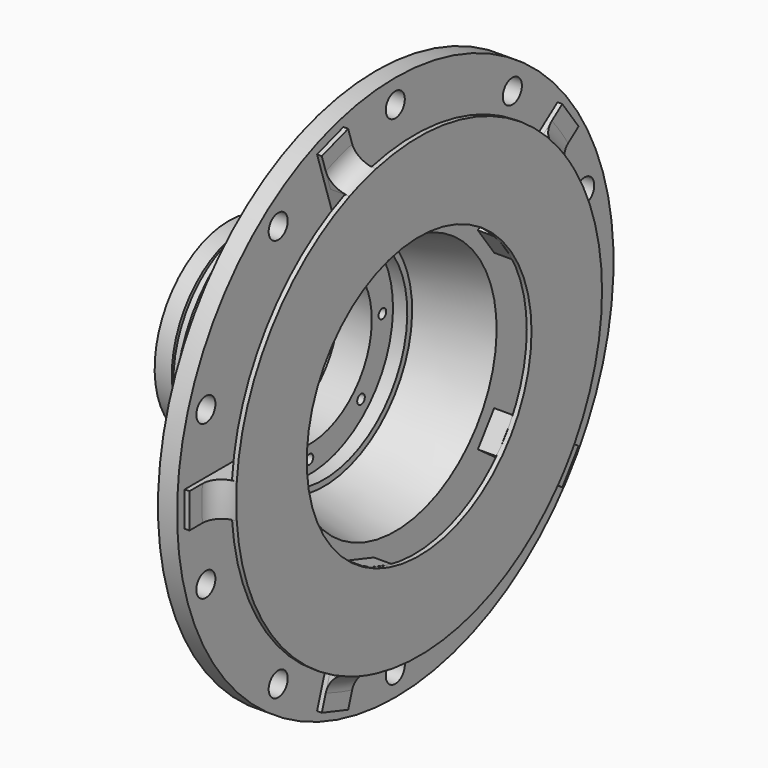
from build123d import *

# Parameters (mm, degrees)
F2_R          = 12.5
F3_DEPTH      = 20
F4_R          = 5
F5_DEPTH      = 20
F6_W          = 129.0251463652
F6_H          = 36.3384204739
F7_DEPTH      = 20
F9_DEPTH      = 5
F10_DEPTH     = 15
F11_T4_ANGLE  = 32.5973484346
F11_T10_ANGLE = 32.5973484346
F11_T16_ANGLE = 32.5973484346
F11_T22_ANGLE = 32.5973484346
F11_T28_ANGLE = 32.5973484346


# Not quite as in the source:
# - a fillet or chamfer that OpenCascade refuses, or shapes differently, is made with other operations: its cross-section is extruded or revolved along the edge and cut away or added


with BuildPart() as f1:
    # F0 (on Front) → F1 (revolve)
    with BuildSketch(Plane.XZ):
        with BuildLine():
            Line((-16.3140908403, 189.203946461), (-16.3140908403, 151.1775321185))
            Line((-16.3140908403, 151.1775321185), (-41.3140908403, 136.1826956272))
            Line((-41.3140908403, 136.1826956272), (-41.3140908403, 124.7942986206))
            Line((-41.3140908403, 124.7942986206), (-111.3140908403, 106.3929200172))
            Line((-111.3140908403, 106.3929200172), (-110.7086323423, 106.3929200172))
            Line((-110.7086323423, 106.3929200172), (-110.7086323423, 103.5716161132))
            Line((-110.7086323423, 103.5716161132), (-117.2448031826, 103.5716161132))
            Line((-117.2448031826, 103.5716161132), (-117.2448031826, 100.1479104161))
            Line((-117.2448031826, 100.1479104161), (-110.7086323423, 100.1479104161))
            Line((-110.7086323423, 100.1479104161), (-110.7086323423, 94.2342355847))
            Line((-110.7086323423, 94.2342355847), (-117.2448031826, 94.2342355847))
            Line((-117.2448031826, 94.2342355847), (-117.2448031826, 82.7181264758))
            Line((-117.2448031826, 82.7181264758), (-123.3140908403, 76.9600793719))
            Line((-123.3140908403, 76.9600793719), (-141.3140908403, 76.9600793719))
            Line((-141.3140908403, 76.9600793719), (-148.0058894081, 70.7351565361))
            Line((-148.0058894081, 70.7351565361), (-165.9934520721, 70.7351565361))
            Line((-165.9934520721, 70.7351565361), (-165.9934520721, 41.6837670207))
            Line((-165.9934520721, 41.6837670207), (-147.6857364697, 41.6837670207))
            Line((-147.6857364697, 41.6837670207), (-138.2742375655, 47.9580983818))
            Line((-138.2742375655, 47.9580983818), (-124.5491505189, 47.9580983818))
            Line((-124.5491505189, 47.9580983818), (-116.3140908403, 55.3639903963))
            Line((-116.3140908403, 55.3639903963), (-81.3140908403, 55.3639903963))
            Line((-81.3140908403, 55.3639903963), (-81.3140908403, 83.1748159732))
            Line((-81.3140908403, 83.1748159732), (-66.3140908403, 83.1748159732))
            Line((-66.3140908403, 83.1748159732), (-66.3140908403, 89.5191647847))
            Line((-66.3140908403, 89.5191647847), (8.6859091597, 106.4794477311))
            Line((8.6859091597, 106.4794477311), (8.6859091597, 259.7348150386))
            Line((8.6859091597, 259.7348150386), (-11.3140908403, 259.7348150386))
            Line((-11.3140908403, 259.7348150386), (-11.3140908403, 209.7348150386))
            Line((-11.3140908403, 209.7348150386), (-41.3140908403, 209.7348150386))
            Line((-41.3140908403, 209.7348150386), (-41.3140908403, 203.7348150386))
            Line((-41.3140908403, 203.7348150386), (-23.6449593669, 198.8411523412))
            ThreePointArc((-23.6449593669, 198.8411523412), (-18.355092325, 195.25822946), (-16.3140908403, 189.203946461))
        make_face()
    revolve(axis=Axis((-78.6537714562, 0, -26.3162329793), (-1, 0, 0)))

    # F2 (on face) → F3 (cut)
    with BuildSketch(Plane(origin=(-11.3140908403, 0, 0), x_dir=(0, -1, 0), z_dir=(-1, 0, 0))):
        with Locations((0, 234.7348150386)):
            Circle(F2_R)
        with Locations((-153.4419561204, 184.8785012666)):
            Circle(F2_R)
        with Locations((-248.2743003031, 54.3529772576)):
            Circle(F2_R)
        with Locations((-248.2743003031, -106.9854432162)):
            Circle(F2_R)
        with Locations((-153.4419561204, -237.5109672252)):
            Circle(F2_R)
        with Locations((0, -287.3672809972)):
            Circle(F2_R)
        with Locations((153.4419561204, -237.5109672252)):
            Circle(F2_R)
        with Locations((248.2743003031, -106.9854432162)):
            Circle(F2_R)
        with Locations((248.2743003031, 54.3529772576)):
            Circle(F2_R)
        with Locations((153.4419561204, 184.8785012666)):
            Circle(F2_R)
    extrude(amount=-F3_DEPTH, mode=Mode.SUBTRACT)

    # F4 (on face) → F5 (cut)
    with BuildSketch(Plane.YZ.offset(-81.3140908403)):
        with Locations((0, 69.2694031847)):
            Circle(F4_R)
        with Locations((-67.5892515156, 41.2730185363)):
            Circle(F4_R)
        with Locations((-95.585636164, -26.3162329793)):
            Circle(F4_R)
        with Locations((-67.5892515156, -93.9054844949)):
            Circle(F4_R)
        with Locations((0, -121.9018691433)):
            Circle(F4_R)
        with Locations((67.5892515156, -93.9054844949)):
            Circle(F4_R)
        with Locations((95.585636164, -26.3162329793)):
            Circle(F4_R)
        with Locations((67.5892515156, 41.2730185363)):
            Circle(F4_R)
    extrude(amount=-F5_DEPTH, mode=Mode.SUBTRACT)

    # F6 (on face) → F7 (join)
    with BuildSketch(Plane.YZ.offset(8.6859091597)):
        with Locations((-211.5166261792, -26.3162329793)):
            Rectangle(F6_W, F6_H)
        Polygon((-102.5776593383, -283.2210069825), (-68.0177677547, -294.4501964577), (-28.1468048262, -171.7399902411), (-62.7066964097, -160.510800766), align=None)
        Polygon((212.6327194043, -203.2613254223), (233.9919070505, -173.8629257102), (129.6083709393, -98.0238475019), (108.2491832932, -127.422247214), align=None)
        Polygon((233.9919070505, 121.2304597516), (212.6327194043, 150.6288594637), (108.2491832932, 74.7897812554), (129.6083709393, 45.3913815433), align=None)
        Polygon((-68.0177677547, 241.8177304991), (-102.5776593383, 230.5885410239), (-62.7066964097, 107.8783348074), (-28.1468048262, 119.1075242825), align=None)
    extrude(amount=F7_DEPTH)

    # F8 (on face) → F9 (join)
    with BuildSketch(Plane.YZ.offset(28.6859091597)):
        with BuildLine():
            Line((-147.0040529966, -8.1470227424), (-239.0119979178, -8.1470227424))
            ThreePointArc((-239.0119979178, -8.1470227424), (-239.701596468, -26.3162329793), (-239.0119979178, -44.4854432162))
            Line((-239.0119979178, -44.4854432162), (-147.0040529966, -44.4854432162))
            Line((-147.0040529966, -44.4854432162), (-147.0040529966, -35.9564862394))
            ThreePointArc((-147.0040529966, -35.9564862394), (-147.3198088526, -26.3162329793), (-147.0040529966, -16.6759797192))
            Line((-147.0040529966, -16.6759797192), (-147.0040529966, -8.1470227424))
        make_face()
        with BuildLine():
            ThreePointArc((-239.0119979178, -44.4854432162), (9.0911460608, -265.8453677679), (239.701596468, -26.3162329793))
            ThreePointArc((239.701596468, -26.3162329793), (9.0911460608, 213.2129018093), (-239.0119979178, -8.1470227424))
            Line((-239.0119979178, -8.1470227424), (-147.0040529966, -8.1470227424))
            Line((-147.0040529966, -8.1470227424), (-147.0040529966, -16.6759797192))
            ThreePointArc((-147.0040529966, -16.6759797192), (4.8227114956, 120.9246157489), (147.3198088526, -26.3162329793))
            ThreePointArc((147.3198088526, -26.3162329793), (4.8227114956, -173.5570817074), (-147.0040529966, -35.9564862394))
            Line((-147.0040529966, -35.9564862394), (-147.0040529966, -44.4854432162))
            Line((-147.0040529966, -44.4854432162), (-239.0119979178, -44.4854432162))
        make_face()
    extrude(amount=F9_DEPTH)

    # F10 (cut): faces of the model
    f10_faces = [f1.faces().sort_by_distance(p)[0] for p in [
        (28.6859091597, -79.6491158165, -271.4510054782),
        (28.6859091597, -257.7499531299, -26.3162329793),
        (28.6859091597, 208.5240923814, -177.8178542081),
        (28.6859091597, -79.6491158165, 218.8185395196),
        (28.6859091597, 208.5240923814, 125.1853882495),
    ]]
    extrude(f10_faces, amount=-F10_DEPTH, mode=Mode.SUBTRACT)

    # F11: fillet of radius 20 on 5 edges, made by hand


with BuildPart() as f11_tool2:
    # F11_s3 → F11_t4 (revolve)
    with BuildSketch(Plane(origin=(0, -7.0886957411, -24.2435313329), x_dir=(1, 0, 0), z_dir=(0, 0.2806444996, 0.9598117861))):
        with BuildLine():
            ThreePointArc((13.6859091597, -252.3160904308), (19.5437735359, -238.1739548071), (33.6859091597, -232.3160904308))
            Line((33.6859091597, -232.3160904308), (33.6859091597, -231.9160904308))
            Line((33.6859091597, -231.9160904308), (13.2859091597, -231.9160904308))
            Line((13.2859091597, -231.9160904308), (13.2859091597, -252.3160904308))
            Line((13.2859091597, -252.3160904308), (13.6859091597, -252.3160904308))
        make_face()
    revolve(axis=Axis((13.6859091597, 0, -26.3162329793), (1, 0, 0)), revolution_arc=F11_T4_ANGLE)

    split(bisect_by=Plane.XY.offset(-44.4854432162), keep=Keep.TOP)

    split(bisect_by=Plane.XY.offset(-8.1470227424), keep=Keep.BOTTOM)


with BuildPart() as f1_1:
    add(f1.part)

    # F11_t1: union F11_tool2
    add(f11_tool2.part)


with BuildPart() as f11_tool8:
    # F11_s9 → F11_t10 (revolve)
    with BuildSketch(Plane(origin=(0, -0.7809680379, -0.0231966772), x_dir=(1, 0, 0), z_dir=(0, 0.9995591734, 0.0296893732))):
        with BuildLine():
            ThreePointArc((13.6859091597, -233.3969643843), (19.5437735359, -219.2548287605), (33.6859091597, -213.3969643843))
            Line((33.6859091597, -213.3969643843), (33.6859091597, -212.9969643843))
            Line((33.6859091597, -212.9969643843), (13.2859091597, -212.9969643843))
            Line((13.2859091597, -212.9969643843), (13.2859091597, -233.3969643843))
            Line((13.2859091597, -233.3969643843), (13.6859091597, -233.3969643843))
        make_face()
    revolve(axis=Axis((13.6859091597, 0, -26.3162329793), (1, 0, 0)), revolution_arc=F11_T10_ANGLE)

    split(bisect_by=Plane(origin=(0, 9.5457989712, 3.101618102), x_dir=(1, 0, 0), z_dir=(0, -0.9510565163, -0.3090169944)), keep=Keep.TOP)

    split(bisect_by=Plane(origin=(0, -25.0140926123, -8.1275713731), x_dir=(1, 0, 0), z_dir=(0, 0.9510565163, 0.3090169944)), keep=Keep.TOP)


with BuildPart() as f1_2:
    add(f1_1.part)

    # F11_t7: union F11_tool8
    add(f11_tool8.part)


with BuildPart() as f11_tool14:
    # F11_s15 → F11_t16 (revolve)
    with BuildSketch(Plane(origin=(0, 12.2507186828, -8.3564583064), x_dir=(1, 0, 0), z_dir=(0, -0.8261113339, 0.5635069335))):
        with BuildLine():
            ThreePointArc((13.6859091597, -281.4417347966), (19.5437735359, -267.2995991729), (33.6859091597, -261.4417347966))
            Line((33.6859091597, -261.4417347966), (33.6859091597, -261.0417347966))
            Line((33.6859091597, -261.0417347966), (13.2859091597, -261.0417347966))
            Line((13.2859091597, -261.0417347966), (13.2859091597, -281.4417347966))
            Line((13.2859091597, -281.4417347966), (13.6859091597, -281.4417347966))
        make_face()
    revolve(axis=Axis((13.6859091597, 0, -26.3162329793), (1, 0, 0)), revolution_arc=F11_T16_ANGLE)

    split(bisect_by=Plane(origin=(0, 25.0140926123, -8.1275713731), x_dir=(1, 0, 0), z_dir=(0, -0.9510565163, 0.3090169944)), keep=Keep.TOP)

    split(bisect_by=Plane(origin=(0, -9.5457989712, 3.101618102), x_dir=(1, 0, 0), z_dir=(0, 0.9510565163, -0.3090169944)), keep=Keep.TOP)


with BuildPart() as f1_3:
    add(f1_2.part)

    # F11_t13: union F11_tool14
    add(f11_tool14.part)


with BuildPart() as f11_tool20:
    # F11_s21 → F11_t22 (revolve)
    with BuildSketch(Plane(origin=(0, 8.3523285705, -23.3254483425), x_dir=(1, 0, 0), z_dir=(0, 0.3371170433, -0.9414627444))):
        with BuildLine():
            ThreePointArc((13.6859091597, -250.8299458158), (19.5437735359, -236.6878101921), (33.6859091597, -230.8299458158))
            Line((33.6859091597, -230.8299458158), (33.6859091597, -230.4299458158))
            Line((33.6859091597, -230.4299458158), (13.2859091597, -230.4299458158))
            Line((13.2859091597, -230.4299458158), (13.2859091597, -250.8299458158))
            Line((13.2859091597, -250.8299458158), (13.6859091597, -250.8299458158))
        make_face()
    revolve(axis=Axis((13.6859091597, 0, -26.3162329793), (1, 0, 0)), revolution_arc=F11_T22_ANGLE)

    split(bisect_by=Plane(origin=(0, 1.8345186066, -2.5249982429), x_dir=(1, 0, 0), z_dir=(0, 0.5877852523, -0.8090169944)), keep=Keep.TOP)

    split(bisect_by=Plane(origin=(0, 23.1937062527, -31.923397955), x_dir=(1, 0, 0), z_dir=(0, -0.5877852523, 0.8090169944)), keep=Keep.TOP)


with BuildPart() as f1_4:
    add(f1_3.part)

    # F11_t19: union F11_tool20
    add(f11_tool20.part)


with BuildPart() as f11_tool26:
    # F11_s27 → F11_t28 (revolve)
    with BuildSketch(Plane(origin=(0, -12.7333834744, -9.8419477893), x_dir=(1, 0, 0), z_dir=(0, -0.7912093825, -0.6115453484))):
        with BuildLine():
            ThreePointArc((13.6859091597, -280.5232469123), (19.5437735359, -266.3811112886), (33.6859091597, -260.5232469123))
            Line((33.6859091597, -260.5232469123), (33.6859091597, -260.1232469123))
            Line((33.6859091597, -260.1232469123), (13.2859091597, -260.1232469123))
            Line((13.2859091597, -260.1232469123), (13.2859091597, -280.5232469123))
            Line((13.2859091597, -280.5232469123), (13.6859091597, -280.5232469123))
        make_face()
    revolve(axis=Axis((13.6859091597, 0, -26.3162329793), (1, 0, 0)), revolution_arc=F11_T28_ANGLE)

    split(bisect_by=Plane(origin=(0, -23.1937062527, -31.923397955), x_dir=(1, 0, 0), z_dir=(0, 0.5877852523, 0.8090169944)), keep=Keep.TOP)

    split(bisect_by=Plane(origin=(0, -1.8345186066, -2.5249982429), x_dir=(1, 0, 0), z_dir=(0, -0.5877852523, -0.8090169944)), keep=Keep.TOP)


with BuildPart() as f1_5:
    add(f1_4.part)

    # F11_t25: union F11_tool26
    add(f11_tool26.part)


solid = f1_5.part
